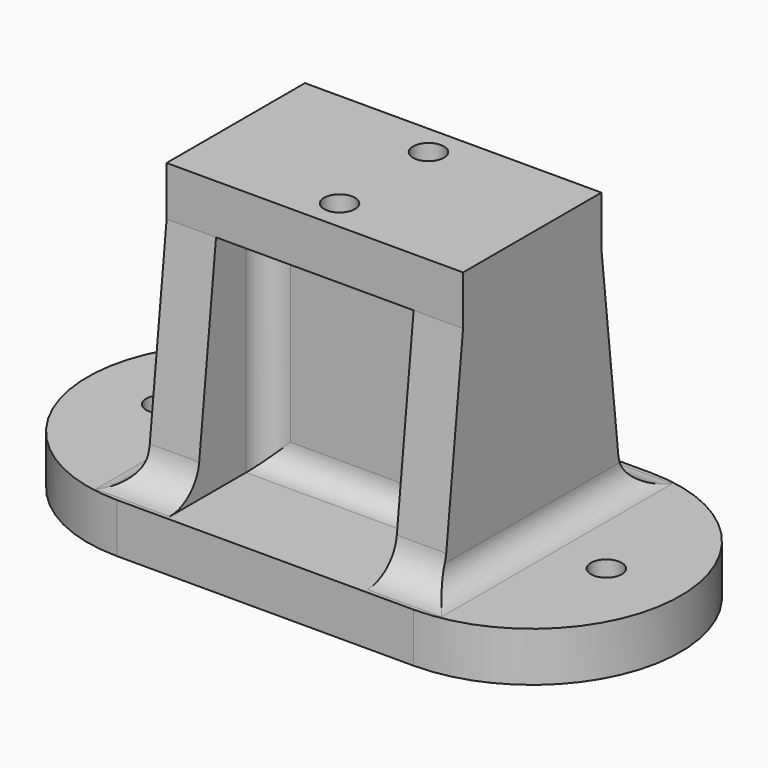
from build123d import *

# Parameters (mm, degrees)
F1_DEPTH  = 12.7
F3_DEPTH  = 38.1
F5_DEPTH  = 25.4
F7_DEPTH  = 12.7
F9_DEPTH  = 12.7
F10_R     = 3.96875
F11_DEPTH = 25.4
F12_DEPTH = 82.551
F13_R     = 9.525
F14_R     = 6.35


# Not quite as in the source:
# - a length typed as a fraction of an inch, garbled in the dataset ("3 / 203.2 mm" for 3/8 in), is restored


with BuildPart() as f1:
    # F0 (on Top) → F1 (new body)
    with BuildSketch(Plane.XY):
        with BuildLine():
            Line((-38.1, -38.1), (38.1, -38.1))
            ThreePointArc((38.1, -38.1), (76.2, 0), (38.1, 38.1))
            Line((38.1, 38.1), (-38.1, 38.1))
            ThreePointArc((-38.1, 38.1), (-76.2, 0), (-38.1, -38.1))
        make_face()
    extrude(amount=F1_DEPTH)

    # F2 (on Right) → F3 (join, symmetric)
    with BuildSketch(Plane.YZ):
        Polygon((6.4445460903, 82.55), (0, 82.55), (-6.2554539097, 82.55), (-22.225, 82.55), (-22.225, 69.85), (-6.2554539097, 69.85), (-6.2554539097, 0), (6.4445460903, 0), (6.4445460903, 69.85), (22.225, 69.85), (22.225, 82.55), align=None)
    extrude(amount=F3_DEPTH, both=True)

    # F4 (on face) → F5 (cut)
    with BuildSketch(Plane.XZ.offset(6.2554539097)):
        with BuildLine():
            Line((7.9375, 69.85), (-7.9375, 69.85))
            ThreePointArc((-7.9375, 69.85), (0, 61.9125), (7.9375, 69.85))
        make_face()
    extrude(amount=-F5_DEPTH, mode=Mode.SUBTRACT)

    # F6 (on face) → F7 (join)
    with BuildSketch(Plane.YZ.offset(38.1)):
        Polygon((-28.575, 12.7), (28.575, 12.7), (22.225, 69.85), (-22.225, 69.85), align=None)
    extrude(amount=-F7_DEPTH)

    # F8 (on face) → F9 (join)
    with BuildSketch(Plane(origin=(-38.1, 0, 0), x_dir=(0, -1, 0), z_dir=(-1, 0, 0))):
        Polygon((-22.225, 69.85), (-28.575, 12.6521781883), (28.575, 12.6521781883), (22.225, 69.85), align=None)
    extrude(amount=-F9_DEPTH)

    # F10 (on face) → F11 (cut)
    with BuildSketch(Plane.XY.offset(82.55)):
        with Locations((0, 14.2875)):
            Circle(F10_R)
        with Locations((0, -14.2875)):
            Circle(F10_R)
    extrude(amount=-F11_DEPTH, mode=Mode.SUBTRACT)

    # F10 (on face) → F12 (cut, through all)
    with BuildSketch(Plane.XY.offset(82.55)):
        with Locations((-57.15, 0)):
            Circle(F10_R)
        with Locations((57.15, 0)):
            Circle(F10_R)
    extrude(amount=-F12_DEPTH, mode=Mode.SUBTRACT)

    # F13
    f13_edges = [f1.edges().sort_by_distance(p)[0] for p in [
        (31.75, -28.575, 12.7),
        (31.75, 28.575, 12.7),
        (-31.75, -28.569691, 12.7),
        (-31.75, 28.569691, 12.7),
    ]]
    fillet(f13_edges, radius=F13_R)

    # F14
    f14_edges = [f1.edges().sort_by_distance(p)[0] for p in [
        (0, 6.444546, 12.7),
        (0, -6.255454, 12.7),
        (-16.66875, -6.255454, 69.85),
        (16.66875, -6.255454, 69.85),
        (-16.66875, 6.444546, 69.85),
        (16.66875, 6.444546, 69.85),
        (38.1, 0, 12.7),
        (-38.1, 0, 12.7),
        (-25.4, 6.444546, 41.275),
        (25.4, 6.444546, 41.275),
        (-25.4, -6.255454, 41.275),
        (25.4, -6.255454, 41.275),
    ]]
    fillet(f14_edges, radius=F14_R)


solid = f1.part
